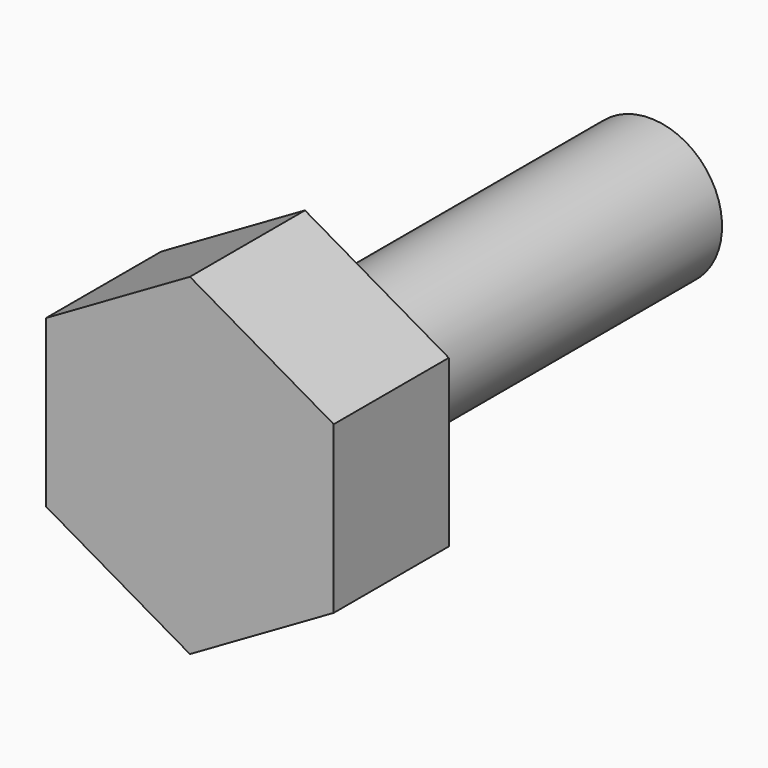
from build123d import *

# Parameters (mm, degrees)
F0_R     = 1
F1_DEPTH = 2
F2_R     = 1
F3_DEPTH = 6


# Not quite as in the source:
# - a feature of the source that left no trace in its solid (it failed there, or was rolled back) is left out


with BuildPart() as f1:
    # F0 (on Front) → F1 (new body)
    with BuildSketch(Plane.XZ):
        Polygon((-2, 1.1547005384), (-2, -1.1547005384), (0, -2.3094010768), (2, -1.1547005384), (2, 1.1547005384), (0, 2.3094010768), align=None)
        Circle(F0_R, mode=Mode.SUBTRACT)
        Circle(F0_R)
    extrude(amount=F1_DEPTH)

    # F2 (on face) → F3 (join)
    with BuildSketch(Plane(origin=(0, 0, 0), x_dir=(-1, 0, 0), z_dir=(0, 1, 0))):
        Circle(F2_R)
    extrude(amount=F3_DEPTH)


solid = f1.part
